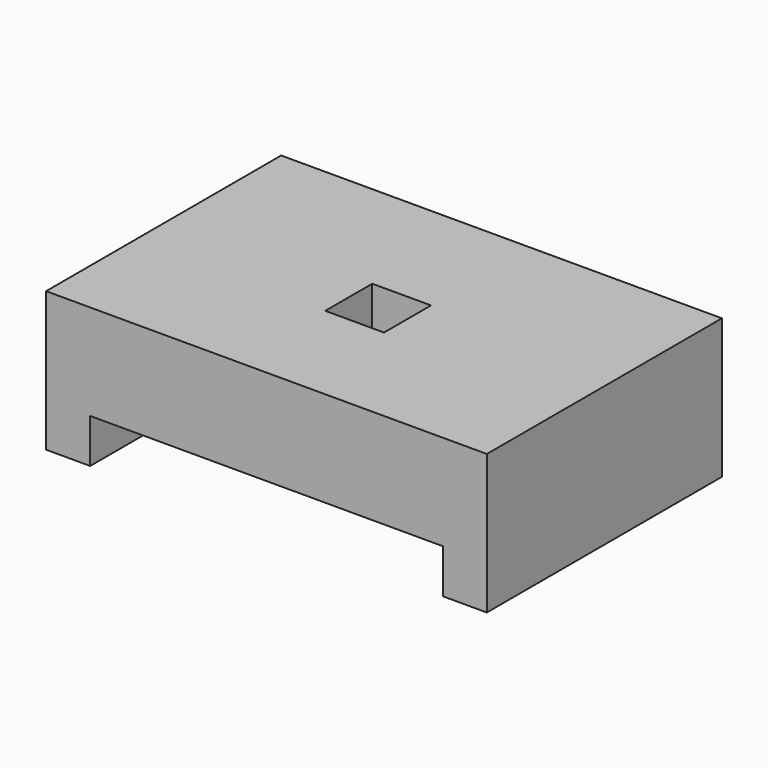
from build123d import *

# Parameters (mm, degrees)
F0_W     = 3
F0_H     = 20
F1_DEPTH = 6.5
F2_DEPTH = 3
F3_DEPTH = 3


# Not quite as in the source:
# - a feature names something its author has since deleted; it is built from what else it names


with BuildPart() as f1:
    # F0 (on Top) → F1 (new body)
    with BuildSketch(Plane.XY):
        with Locations((-1.5, 10)):
            Rectangle(F0_W, F0_H)
        Polygon((-27, 0), (-3, 0), (-3, 20), (-15, 20), (-27, 20), align=None)
        with BuildLine():
            Line((-17, 11.5), (-15, 11.5))
            Line((-15, 11.5), (-13, 11.5))
            Line((-13, 11.5), (-11.5, 11.5))
            ThreePointArc((-11.5, 11.5), (-10.0857864376, 10.9142135624), (-9.5, 9.5))
            ThreePointArc((-9.5, 9.5), (-10.0857864376, 8.0857864376), (-11.5, 7.5))
            Line((-11.5, 7.5), (-13, 7.5))
            Line((-13, 7.5), (-17, 7.5))
            Line((-17, 7.5), (-18.5, 7.5))
            ThreePointArc((-18.5, 7.5), (-20.5, 9.5), (-18.5, 11.5))
            Line((-18.5, 11.5), (-17, 11.5))
        make_face(mode=Mode.SUBTRACT)
        with Locations((-28.5, 10)):
            Rectangle(F0_W, F0_H)
        with BuildLine():
            Line((-17, 10.8228756555), (-17, 11.5))
            Line((-17, 11.5), (-18.5, 11.5))
            ThreePointArc((-18.5, 11.5), (-17.6771243445, 11.3228756555), (-17, 10.8228756555))
        make_face()
        with BuildLine():
            Line((-11.5, 11.5), (-13, 11.5))
            Line((-13, 11.5), (-13, 10.8228756555))
            ThreePointArc((-13, 10.8228756555), (-12.3228756555, 11.3228756555), (-11.5, 11.5))
        make_face()
        with BuildLine():
            ThreePointArc((-17, 10.8228756555), (-17.6771243445, 11.3228756555), (-18.5, 11.5))
            ThreePointArc((-18.5, 11.5), (-20.5, 9.5), (-18.5, 7.5))
            Line((-18.5, 7.5), (-17, 7.5))
            Line((-17, 7.5), (-17, 9.5))
            Line((-17, 9.5), (-17, 10.8228756555))
        make_face()
        with BuildLine():
            ThreePointArc((-9.5, 9.5), (-10.0857864376, 10.9142135624), (-11.5, 11.5))
            ThreePointArc((-11.5, 11.5), (-12.3228756555, 11.3228756555), (-13, 10.8228756555))
            Line((-13, 10.8228756555), (-13, 8.1771243445))
            ThreePointArc((-13, 8.1771243445), (-12.3228756555, 7.6771243445), (-11.5, 7.5))
            ThreePointArc((-11.5, 7.5), (-10.0857864376, 8.0857864376), (-9.5, 9.5))
        make_face()
        with BuildLine():
            ThreePointArc((-11.5, 7.5), (-12.3228756555, 7.6771243445), (-13, 8.1771243445))
            Line((-13, 8.1771243445), (-13, 7.5))
            Line((-13, 7.5), (-11.5, 7.5))
        make_face()
    extrude(amount=F1_DEPTH)

    # F0 (on Top) → F2 (join)
    with BuildSketch(Plane.XY):
        with Locations((-1.5, 10)):
            Rectangle(F0_W, F0_H)
        with Locations((-28.5, 10)):
            Rectangle(F0_W, F0_H)
        with BuildLine():
            Line((-17, 10.8228756555), (-17, 11.5))
            Line((-17, 11.5), (-18.5, 11.5))
            ThreePointArc((-18.5, 11.5), (-17.6771243445, 11.3228756555), (-17, 10.8228756555))
        make_face()
        with BuildLine():
            Line((-11.5, 11.5), (-13, 11.5))
            Line((-13, 11.5), (-13, 10.8228756555))
            ThreePointArc((-13, 10.8228756555), (-12.3228756555, 11.3228756555), (-11.5, 11.5))
        make_face()
        with BuildLine():
            ThreePointArc((-17, 10.8228756555), (-17.6771243445, 11.3228756555), (-18.5, 11.5))
            ThreePointArc((-18.5, 11.5), (-20.5, 9.5), (-18.5, 7.5))
            Line((-18.5, 7.5), (-17, 7.5))
            Line((-17, 7.5), (-17, 9.5))
            Line((-17, 9.5), (-17, 10.8228756555))
        make_face()
        with BuildLine():
            ThreePointArc((-9.5, 9.5), (-10.0857864376, 10.9142135624), (-11.5, 11.5))
            ThreePointArc((-11.5, 11.5), (-12.3228756555, 11.3228756555), (-13, 10.8228756555))
            Line((-13, 10.8228756555), (-13, 8.1771243445))
            ThreePointArc((-13, 8.1771243445), (-12.3228756555, 7.6771243445), (-11.5, 7.5))
            ThreePointArc((-11.5, 7.5), (-10.0857864376, 8.0857864376), (-9.5, 9.5))
        make_face()
        with BuildLine():
            ThreePointArc((-11.5, 7.5), (-12.3228756555, 7.6771243445), (-13, 8.1771243445))
            Line((-13, 8.1771243445), (-13, 7.5))
            Line((-13, 7.5), (-11.5, 7.5))
        make_face()
    extrude(amount=-F2_DEPTH)

    # F0 (on Top) → F3 (join)
    with BuildSketch(Plane.XY):
        with Locations((-28.5, 10)):
            Rectangle(F0_W, F0_H)
        with Locations((-1.5, 10)):
            Rectangle(F0_W, F0_H)
    extrude(amount=-F3_DEPTH)


solid = f1.part
